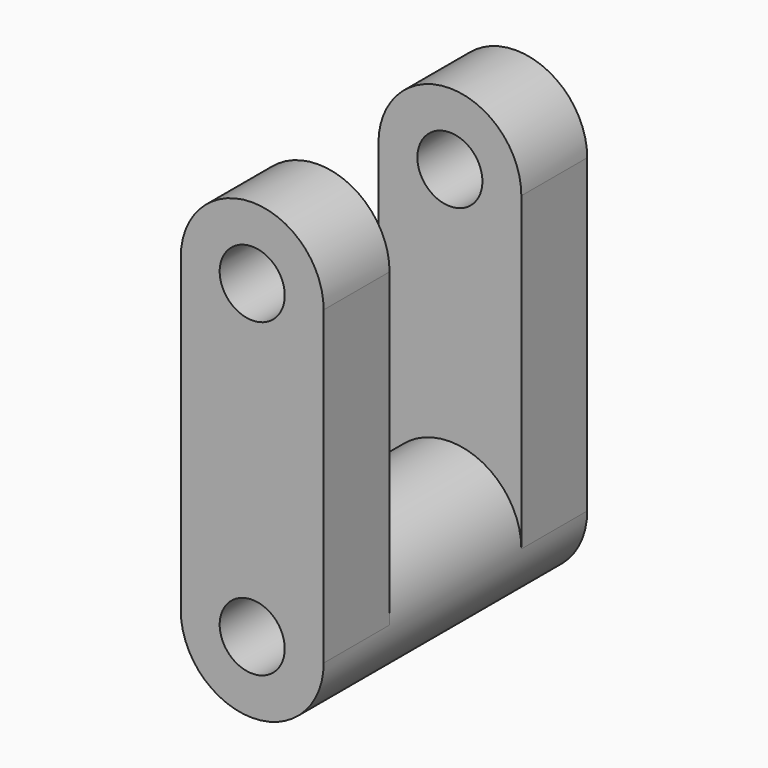
from build123d import *

# Parameters (mm, degrees)
F0_R     = 9.8737284495
F1_DEPTH = 25
F4_R     = 9.8737284495
F5_DEPTH = 50


with BuildPart() as f1:
    # F0 (on Front) → F1 (new body)
    with BuildSketch(Plane.XZ):
        with BuildLine():
            Line((-21.6877176851, 94.382122159), (-21.6877176851, 0))
            ThreePointArc((-21.6877176851, 0), (0, -21.6877176851), (21.6877176851, 0))
            Line((21.6877176851, 0), (21.6877176851, 94.382122159))
            ThreePointArc((21.6877176851, 94.382122159), (0, 116.0698398441), (-21.6877176851, 94.382122159))
        make_face()
        Circle(F0_R, mode=Mode.SUBTRACT)
        with Locations((0, 94.382122159)):
            Circle(F0_R, mode=Mode.SUBTRACT)
    extrude(amount=F1_DEPTH)


with BuildPart() as f3_1:
    # F3: instance of F1
    add(f1.part.mirror(Plane.XZ.offset(50)))


with BuildPart() as f1_1:
    add(f1.part)

    add(f3_1.part)  # F5 merges F3_1
    # F4 (on face) → F5 (join, through all)
    with BuildSketch(Plane(origin=(0, -75, 0), x_dir=(-1, 0, 0), z_dir=(0, 1, 0))):
        with BuildLine():
            ThreePointArc((-21.6877176851, 0), (0, -21.6877176851), (21.6877176851, 0))
            ThreePointArc((21.6877176851, 0), (0, 21.6877176851), (-21.6877176851, 0))
        make_face()
        Circle(F4_R, mode=Mode.SUBTRACT)
    extrude(amount=F5_DEPTH)


solid = f1_1.part
